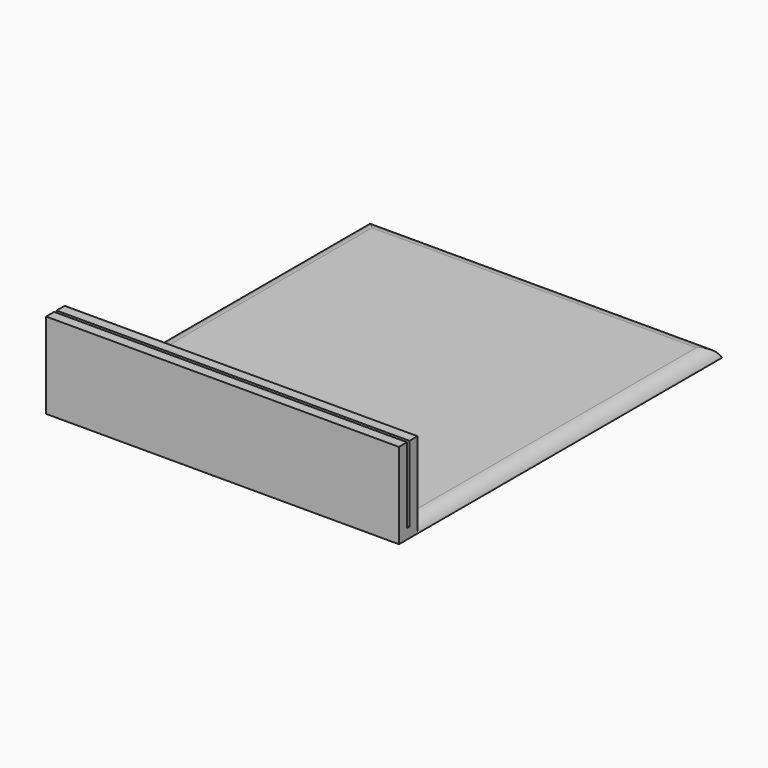
from build123d import *

# Parameters (mm, degrees)
F0_W        = 1.9147001281
F0_H        = 2
F0_W_2      = 0.6
F0_W_3      = 2
F0_H_2      = 15
F0_W_4      = 75.4852998719
F1_DEPTH    = 35
F2_T1_DEPTH = 82.5563676837
F2_T3_DEPTH = 84.1421356237


# Not quite as in the source:
# - a fillet or chamfer that OpenCascade refuses, or shapes differently, is made with other operations: its cross-section is extruded or revolved along the edge and cut away or added


with BuildPart() as f1:
    # F0 (on Right) → F1 (new body, symmetric)
    with BuildSketch(Plane.YZ):
        Polygon((-48.8228555396, -4.8070274784), (-48.8228555396, -2.8070274784), (-46.9081554115, -2.8070274784), (-46.9081554115, 12.1929725216), (-48.9081554115, 12.1929725216), (-48.9081554115, -4.8070274784), align=None)
        with Locations((-47.8655054756, -3.8070274784)):
            Rectangle(F0_W, F0_H)
        with Locations((-46.6081554115, -3.8070274784)):
            Rectangle(F0_W_2, F0_H)
        with Locations((-45.3081554115, 4.6929725216)):
            Rectangle(F0_W_3, F0_H_2)
        with Locations((-45.3081554115, -3.8070274784)):
            Rectangle(F0_W_3, F0_H)
        with Locations((-6.5655054756, -3.8070274784)):
            Rectangle(F0_W_4, F0_H)
    extrude(amount=F1_DEPTH, both=True)

    # F2: fillet of radius 3 on 3 edges, made by hand

    # F2_s2 → F2_t1 (cut)
    with BuildSketch(Plane.XZ.offset(-38.2482122722)):
        with BuildLine():
            ThreePointArc((32.1715728753, -2.8070274784), (33.9036236828, -3.3575377356), (35, -4.8070274784))
            Line((35, -4.8070274784), (35, -2.8070274784))
            Line((35, -2.8070274784), (32.1715728753, -2.8070274784))
        make_face()
        with BuildLine():
            ThreePointArc((-32.1715728753, -2.8070274784), (-33.9036236828, -3.3575377356), (-35, -4.8070274784))
            Line((-35, -4.8070274784), (-35, -2.8070274784))
            Line((-35, -2.8070274784), (-32.1715728753, -2.8070274784))
        make_face()
    extrude(amount=F2_T1_DEPTH, mode=Mode.SUBTRACT)

    # F2_s4 → F2_t3 (cut)
    with BuildSketch(Plane.YZ.offset(-42.0710678119)):
        with BuildLine():
            ThreePointArc((28.3487173356, -2.8070274784), (30.0807681432, -3.3575377356), (31.1771444604, -4.8070274784))
            Line((31.1771444604, -4.8070274784), (31.1771444604, -2.8070274784))
            Line((31.1771444604, -2.8070274784), (28.3487173356, -2.8070274784))
        make_face()
    extrude(amount=F2_T3_DEPTH, mode=Mode.SUBTRACT)


solid = f1.part
